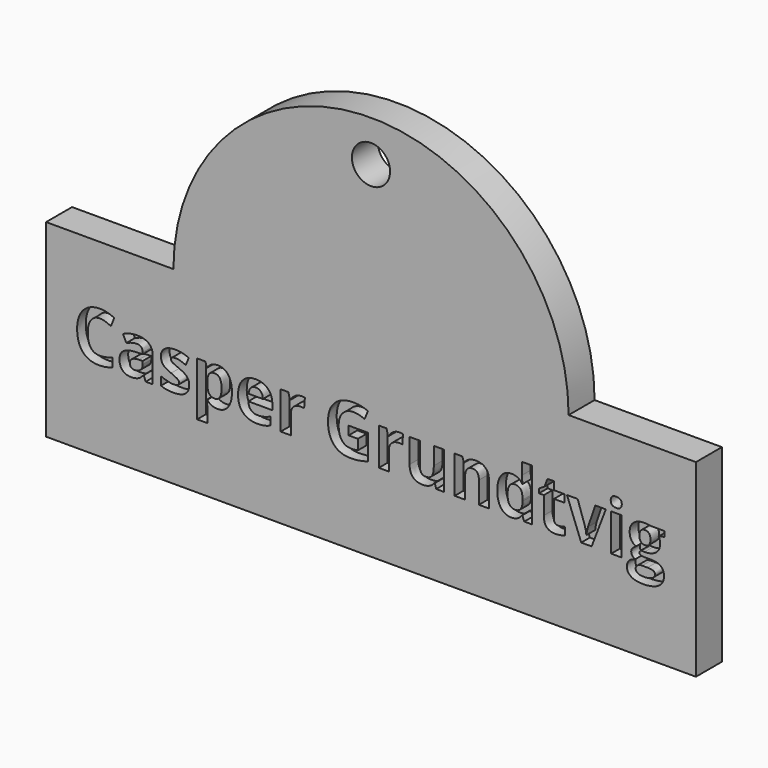
from build123d import *

# Parameters (mm, degrees)
F0_R         = 3.5219274683
F1_DEPTH     = 6
F2_TEXT_SIZE = 12.6040640945
F3_DEPTH     = 2


# Not quite as in the source:
# - Text() gives the source's letters only with a copy of the font that has no kerning and outlines rounded to 1/6400 em; it was checked with that copy


with BuildPart() as f1:
    # F0 (on Front) → F1 (new body)
    with BuildSketch(Plane.XZ):
        with BuildLine():
            Line((-60, -17.4469049121), (60, -17.4469049121))
            Line((60, -17.4469049121), (60, 17.4469049121))
            Line((60, 17.4469049121), (36.4871999276, 17.4469049121))
            ThreePointArc((36.4871999276, 17.4469049121), (0, 53.9341048397), (-36.4871999276, 17.4469049121))
            Line((-36.4871999276, 17.4469049121), (-60, 17.4469049121))
            Line((-60, 17.4469049121), (-60, -17.4469049121))
        make_face()
        with Locations((0, 46.3127195835)):
            Circle(F0_R, mode=Mode.SUBTRACT)
    extrude(amount=F1_DEPTH)

    # F2 (on face) → F3 (cut)
    with BuildSketch(Plane.XZ.offset(6)):
        with Locations((-55, -2.5254925118)):
            Text('Casper Grundtvig', F2_TEXT_SIZE, font='Open Sans', font_style=FontStyle.BOLD, text_align=(TextAlign.LEFT, TextAlign.BOTTOM))
    extrude(amount=-F3_DEPTH, mode=Mode.SUBTRACT)


solid = f1.part
